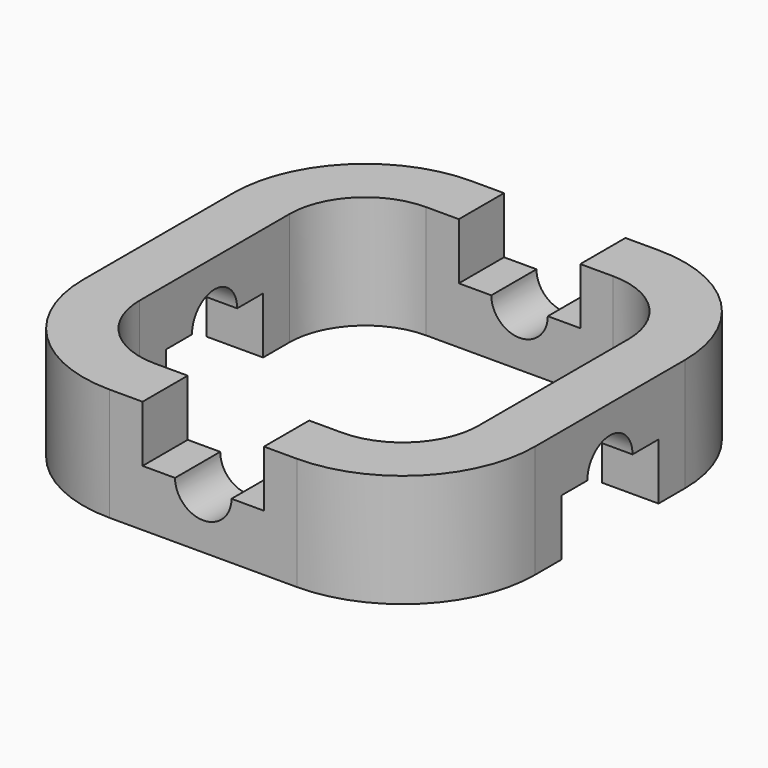
from build123d import *

# Parameters (mm, degrees)
F1_DEPTH      = 40
F2_R          = 10
F3_DEPTH      = 180
F3_DEPTH_BACK = 20
F4_R          = 10
F5_DEPTH      = 20
F5_DEPTH_BACK = 180
F7_DEPTH      = 181.4
F9_DEPTH      = 244.2


# Not quite as in the source:
# - a feature names something its author has since deleted; it is built from what else it names


with BuildPart() as f1:
    # F0 (on Top) → F1 (new body)
    with BuildSketch(Plane.XY):
        with BuildLine():
            Line((-33.1370849898, -80), (33.1370849898, -80))
            ThreePointArc((33.1370849898, -80), (66.2741699797, -66.2741699797), (80, -33.1370849898))
            Line((80, -33.1370849898), (80, 33.1370849898))
            ThreePointArc((80, 33.1370849898), (66.2741699797, 66.2741699797), (33.1370849898, 80))
            Line((33.1370849898, 80), (-33.1370849898, 80))
            ThreePointArc((-33.1370849898, 80), (-66.2741699797, 66.2741699797), (-80, 33.1370849898))
            Line((-80, 33.1370849898), (-80, -33.1370849898))
            ThreePointArc((-80, -33.1370849898), (-66.2741699797, -66.2741699797), (-33.1370849898, -80))
        make_face()
        with BuildLine():
            Line((33.1370849898, -60), (24.8528137424, -60))
            Line((24.8528137424, -60), (-24.8528137424, -60))
            Line((-24.8528137424, -60), (-33.1370849898, -60))
            ThreePointArc((-33.1370849898, -60), (-52.132034356, -52.132034356), (-60, -33.1370849898))
            Line((-60, -33.1370849898), (-60, -24.8528137424))
            Line((-60, -24.8528137424), (-60, 24.8528137424))
            Line((-60, 24.8528137424), (-60, 33.1370849898))
            ThreePointArc((-60, 33.1370849898), (-52.132034356, 52.132034356), (-33.1370849898, 60))
            Line((-33.1370849898, 60), (-24.8528137424, 60))
            Line((-24.8528137424, 60), (24.8528137424, 60))
            Line((24.8528137424, 60), (33.1370849898, 60))
            ThreePointArc((33.1370849898, 60), (52.132034356, 52.132034356), (60, 33.1370849898))
            Line((60, 33.1370849898), (60, 24.8528137424))
            Line((60, 24.8528137424), (60, -24.8528137424))
            Line((60, -24.8528137424), (60, -33.1370849898))
            ThreePointArc((60, -33.1370849898), (52.132034356, -52.132034356), (33.1370849898, -60))
        make_face(mode=Mode.SUBTRACT)
    extrude(amount=F1_DEPTH)

    # F2 (on face) → F3 (cut, two sides)
    with BuildSketch(Plane.XZ.offset(80)) as f3_sk:
        with Locations((0, 20)):
            Circle(F2_R)
    extrude(amount=-F3_DEPTH, mode=Mode.SUBTRACT)
    extrude(f3_sk.sketch, amount=F3_DEPTH_BACK, mode=Mode.SUBTRACT)

    # F4 (on face) → F5 (cut, two sides)
    with BuildSketch(Plane.YZ.offset(80)) as f5_sk:
        with Locations((0, 20)):
            Circle(F4_R)
    extrude(amount=F5_DEPTH, mode=Mode.SUBTRACT)
    extrude(f5_sk.sketch, amount=-F5_DEPTH_BACK, mode=Mode.SUBTRACT)

    # F6 (on face) → F7 (cut)
    with BuildSketch(Plane.XZ.offset(80)):
        Polygon((-21.5, 40), (0, 40), (0, 51.6958795488), (-57.5, 51.6958795488), (-71.9271823764, 52.9654417948), (-71.9271823764, 40), (-59.4264046908, 40), (-33.1370849898, 40), align=None)
        with BuildLine():
            Line((0, 40), (0, 30))
            ThreePointArc((0, 30), (7.0710678119, 27.0710678119), (10, 20))
            Line((10, 20), (21.5, 20))
            Line((21.5, 20), (21.5, 33))
            Line((21.5, 33), (21.5, 40))
            Line((21.5, 40), (0, 40))
        make_face()
        Polygon((0, 51.6958795488), (0, 40), (21.5, 40), (21.5, 45.9314808249), (59.4264046908, 40), (71.9271823764, 40), (71.9271823764, 52.9654417948), (57.5, 51.6958795488), align=None)
        with BuildLine():
            Line((-21.5, 20), (-10, 20))
            ThreePointArc((-10, 20), (-7.0710678119, 27.0710678119), (0, 30))
            Line((0, 30), (0, 40))
            Line((0, 40), (-21.5, 40))
            Line((-21.5, 40), (-21.5, 33))
            Line((-21.5, 33), (-21.5, 20))
        make_face()
    extrude(amount=-F7_DEPTH, mode=Mode.SUBTRACT)

    # F8 (on face) → F9 (cut)
    with BuildSketch(Plane.YZ.offset(80)):
        Polygon((21.5, 0), (0, 0), (0, -11.1064584926), (57.5, -11.1064584926), (66.6687613726, -11.8878306821), (66.6687613726, 0), (59.4264046908, 0), (21.5, -5.7359817438), align=None)
        with BuildLine():
            ThreePointArc((10, 20), (7.0710678119, 12.9289321881), (0, 10))
            Line((0, 10), (0, 0))
            Line((0, 0), (21.5, 0))
            Line((21.5, 0), (21.5, 7))
            Line((21.5, 7), (21.5, 20))
            Line((21.5, 20), (10, 20))
        make_face()
        with BuildLine():
            ThreePointArc((0, 10), (-7.0710678119, 12.9289321881), (-10, 20))
            Line((-10, 20), (-21.5, 20))
            Line((-21.5, 20), (-21.5, 7))
            Line((-21.5, 7), (-21.5, 0))
            Line((-21.5, 0), (0, 0))
            Line((0, 0), (0, 10))
        make_face()
        Polygon((0, -11.1064584926), (0, 0), (-21.5, 0), (-21.5, -3.4078599419), (-59.4264046908, 0), (-66.6687613726, 0), (-66.6687613726, -11.8878306821), (-57.5, -11.1064584926), align=None)
    extrude(amount=-F9_DEPTH, mode=Mode.SUBTRACT)


solid = f1.part
